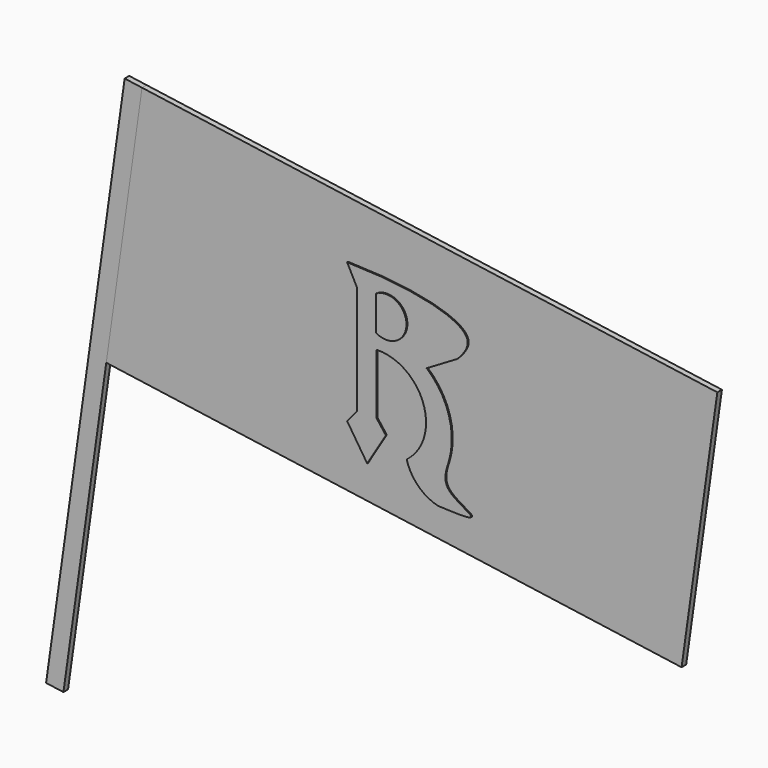
from build123d import *

# Parameters (mm, degrees)
F3_DEPTH = 1.27
F4_DEPTH = 1.524
F5_DEPTH = 1.778
F6_DEPTH = 1.27


with BuildPart() as f3:
    # F0 (on Front) → F3 (new body)
    with BuildSketch(Plane.XZ):
        Polygon((-46.8397970266, 66.7252085961), (-64.2335191369, -56.7155890167), (-60.3914538267, -57.2569644584), (-50.9105029018, 10.0280097917), (-42.9977317164, 66.1838331544), align=None)
    extrude(amount=F3_DEPTH)


with BuildPart() as f4:
    # F1 (on face) → F4 (new body)
    with BuildSketch(Plane.XZ):
        with BuildLine():
            add(Edge.make_bspline(
                [(2.611707896, 47.1022129059), (16.8176115922, 46.8540078192), (30.9562098752, 43.4945430076), (29.3138485804, 38.6144516592), (27.0463850214, 36.2234011264)],
                knots=[0, 0, 0, 0, 0.6865167279, 1, 1, 1, 1], degree=3))
            Line((2.611707896, 47.1022129059), (4.8332214355, 42.8178682923))
            Line((4.8332214355, 42.8178682923), (4.8332214355, 18.8572574407))
            Line((4.8332214355, 18.8572574407), (2.611707896, 16.1597058177))
            Line((2.611707896, 16.1597058177), (7.0547349751, 9.3364855275))
            Line((7.0547349751, 9.3364855275), (11.1804036424, 16.1597058177))
            Line((11.1804036424, 16.1597058177), (9.1175679117, 18.8572574407))
            Line((9.1175679117, 18.8572574407), (9.1175679117, 32.1863368154))
            ThreePointArc((9.1175679117, 32.1863368154), (19.4937940987, 25.0312352135), (15.7821085304, 12.9861142486))
            ThreePointArc((15.7821085304, 12.9861142486), (18.3468119295, 8.6267160163), (22.7640103549, 6.1628948897))
            add(Edge.make_bspline(
                [(25.0928570651, 15.5296488348), (24.4625847415, 13.603531459), (23.1621461709, 9.6293805516), (33.7093394749, 5.701443681), (26.5178697982, 6.0046335018), (22.7640103549, 6.1628948897)],
                knots=[0, 0, 0, 0, 0.3101340133, 0.6398983705, 1, 1, 1, 1], degree=3))
            ThreePointArc((25.0928570651, 15.5296488348), (25.142772253, 24.5838471684), (20.2251356095, 32.1863368154))
            Line((20.2251356095, 32.1863368154), (27.0463850214, 36.2234011264))
        make_face()
    extrude(amount=F4_DEPTH)


with BuildPart() as f5:
    # F2 (on face) → F5 (new body)
    with BuildSketch(Plane.XZ):
        with BuildLine():
            ThreePointArc((9.1935675591, 35.6048643589), (15.9484374114, 39.419779554), (9.1935675591, 43.2346947491))
            Line((9.1935675591, 43.2346947491), (9.1935675591, 35.6048643589))
        make_face()
    extrude(amount=F5_DEPTH)


with BuildPart() as f6:
    # F0 (on Front) → F6 (new body)
    with BuildSketch(Plane.XZ):
        Polygon((84.3527845457, 48.2392027461), (-42.9977317164, 66.1838331544), (-50.9105029018, 10.0280097917), (76.4400133604, -7.9166206166), align=None)
    extrude(amount=F6_DEPTH)


solid = Compound([f3.part, f4.part, f5.part, f6.part])
